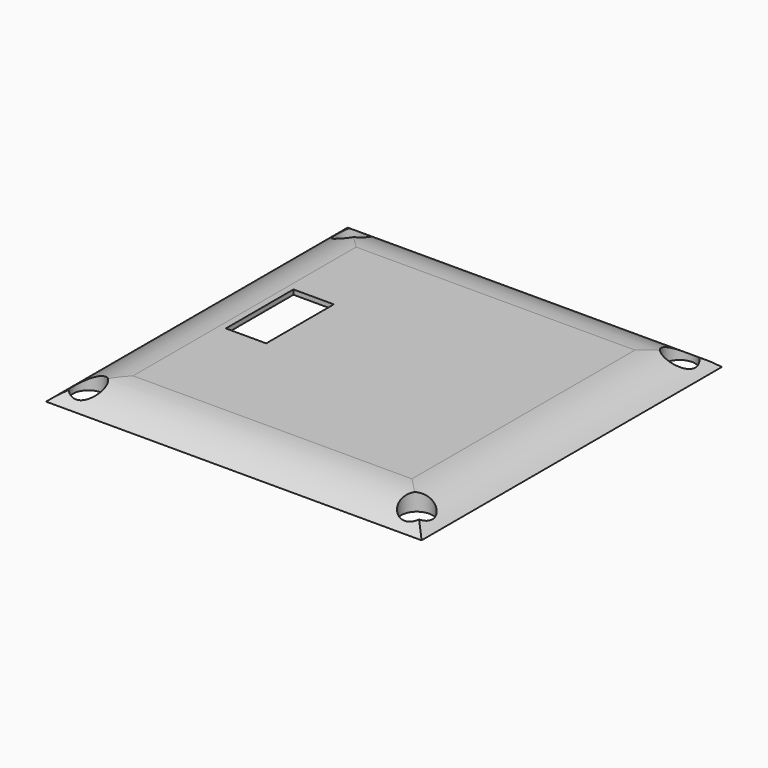
from build123d import *

# Parameters (mm, degrees)
F0_W        = 40
F0_H        = 40
F1_DEPTH    = 2
F2_T1_DEPTH = 65.7293606605
F2_T3_DEPTH = 65.7293606605
F3_D        = 3.3
F4_W        = 4.3
F4_H        = 9
F5_DEPTH    = 25
F6_W        = 32
F6_H        = 32
F7_DEPTH    = 1.5


# Not quite as in the source:
# - a fillet or chamfer that OpenCascade refuses, or shapes differently, is made with other operations: its cross-section is extruded or revolved along the edge and cut away or added


with BuildPart() as f1:
    # F0 (on Top) → F1 (new body)
    with BuildSketch(Plane.XY):
        with Locations((0.9159009159, 13.0545736344)):
            Rectangle(F0_W, F0_H)
    extrude(amount=F1_DEPTH)

    # F2: fillet of radius 7.62 on 4 edges, made by hand

    # F2_s2 → F2_t1 (cut)
    with BuildSketch(Plane.XZ.offset(-45.9192539647)):
        with BuildLine():
            ThreePointArc((-19.0840990841, 0), (-16.6986617004, 1.4824221221), (-13.938226952, 2))
            Line((-13.938226952, 2), (-19.0840990841, 2))
            Line((-19.0840990841, 2), (-19.0840990841, 0))
        make_face()
        with BuildLine():
            ThreePointArc((20.9159009159, 0), (18.5304635321, 1.4824221221), (15.7700287838, 2))
            Line((15.7700287838, 2), (20.9159009159, 2))
            Line((20.9159009159, 2), (20.9159009159, 0))
        make_face()
    extrude(amount=F2_T1_DEPTH, mode=Mode.SUBTRACT)

    # F2_s4 → F2_t3 (cut)
    with BuildSketch(Plane.YZ.offset(-31.9487794144)):
        with BuildLine():
            ThreePointArc((-6.9454263656, 0), (-4.5599889818, 1.4824221221), (-1.7995542335, 2))
            Line((-1.7995542335, 2), (-6.9454263656, 2))
            Line((-6.9454263656, 2), (-6.9454263656, 0))
        make_face()
        with BuildLine():
            ThreePointArc((33.0545736344, 0), (30.6691362507, 1.4824221221), (27.9087015023, 2))
            Line((27.9087015023, 2), (33.0545736344, 2))
            Line((33.0545736344, 2), (33.0545736344, 0))
        make_face()
    extrude(amount=F2_T3_DEPTH, mode=Mode.SUBTRACT)

    # F3 (through all)
    with Locations(Plane(origin=(0, 0, 0), x_dir=(1, 0, 0), z_dir=(0, 0, -1))):
        with Locations((-16.5840990841, 4.4454263656), (-16.5840990841, -30.5545736344), (18.4159009159, -30.5545736344), (18.4159009159, 4.4454263656)):
            Hole(F3_D / 2)

    # F4 (on Top) → F5 (cut)
    with BuildSketch(Plane.XY):
        with Locations((-11.0940990841, 14.1945736344)):
            Rectangle(F4_W, F4_H)
    extrude(amount=F5_DEPTH, mode=Mode.SUBTRACT)

    # F6 (on Top) → F7 (cut)
    with BuildSketch(Plane.XY):
        with Locations((0.9159009159, 13.0545736344)):
            Rectangle(F6_W, F6_H)
    extrude(amount=F7_DEPTH, mode=Mode.SUBTRACT)


solid = f1.part
